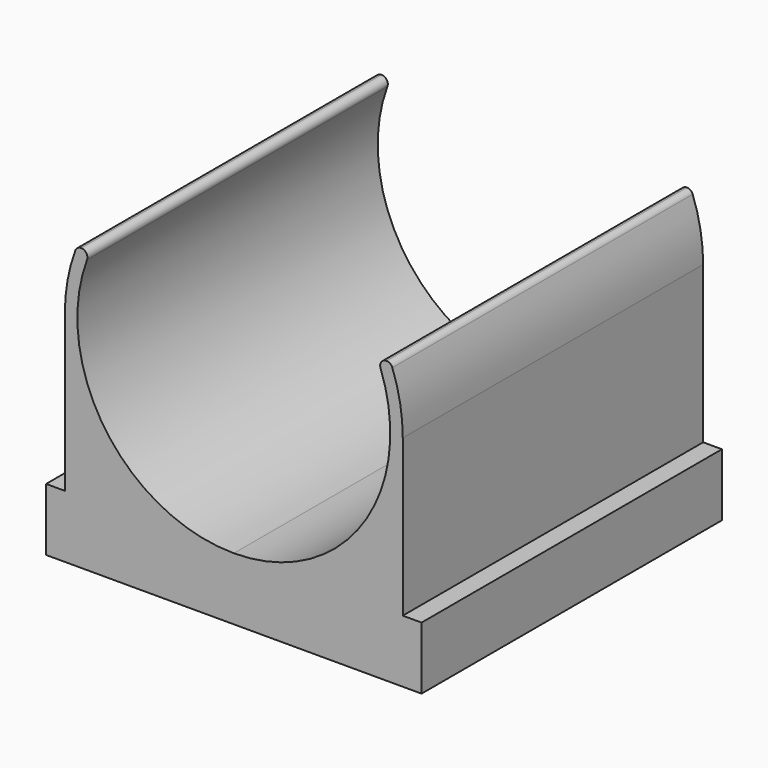
from build123d import *

# Parameters (mm, degrees)
F1_W     = 30
F1_H     = 30
F2_DEPTH = 5
F3_DEPTH = 15
F4_R     = 0.49999


# Not quite as in the source:
# - a fillet or chamfer is up to 0.001 mm smaller than in the source, because OpenCascade refuses the exact size


with BuildPart() as f2:
    # F1 (on Top) → F2 (new body)
    with BuildSketch(Plane.XY):
        Rectangle(F1_W, F1_H)
    extrude(amount=-F2_DEPTH)

    # F0 (on Front) → F3 (join, symmetric)
    with BuildSketch(Plane.XZ):
        with BuildLine():
            ThreePointArc((0, 0), (-10.4582503317, 5.6534680312), (-11.4564392374, 17.5))
            Line((-11.4564392374, 17.5), (-12.539936204, 17.5))
            ThreePointArc((-12.539936204, 17.5), (-13.257811636, 15.0456689932), (-13.5, 12.5))
            Line((-13.5, 12.5), (-13.5, 0))
            Line((-13.5, 0), (0, 0))
        make_face()
        with BuildLine():
            ThreePointArc((11.4564392374, 17.5), (10.4582503317, 5.6534680312), (0, 0))
            Line((0, 0), (13.5, 0))
            Line((13.5, 0), (13.5, 12.5))
            ThreePointArc((13.5, 12.5), (13.257811636, 15.0456689932), (12.539936204, 17.5))
            Line((12.539936204, 17.5), (11.4564392374, 17.5))
        make_face()
    extrude(amount=F3_DEPTH, both=True)

    # F4 (radius 0.5 in the source; OpenCascade refuses exactly that, so slightly less here)
    f4_edges = [f2.edges().sort_by_distance(p)[0] for p in [
        (-11.456439, 0, 17.5),
        (12.539936, 0, 17.5),
        (-12.539936, 0, 17.5),
        (11.456439, 0, 17.5),
    ]]
    fillet(f4_edges, radius=F4_R)


solid = f2.part
